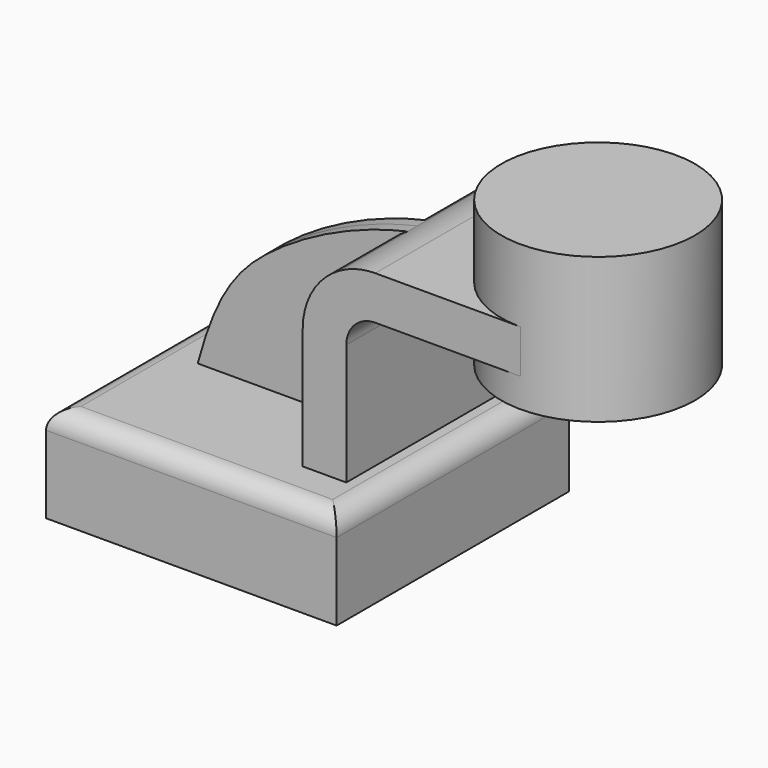
from build123d import *

# Parameters (mm, degrees)
F1_DEPTH = 38.1
F2_DEPTH = 25.4
F4_DEPTH = 3.175
F5_R     = 5.08


with BuildPart() as f1:
    # F0 (on Front) → F1 (new body, symmetric)
    with BuildSketch(Plane.XZ):
        Polygon((38.1, -12.7), (38.1, 12.7), (30.48, 12.7), (19.05, 12.7), (-26.270797, 12.7), (-38.1, 12.7), (-38.1, -12.7), align=None)
    extrude(amount=F1_DEPTH, both=True)

    # F0 (on Front) → F2 (join, symmetric)
    with BuildSketch(Plane.XZ):
        with BuildLine():
            Line((19.05, 12.7), (30.48, 12.7))
            Line((30.48, 12.7), (30.48, 44.45))
            ThreePointArc((30.48, 44.45), (32.711846, 49.838154), (38.1, 52.07))
            Line((38.1, 52.07), (76.2, 52.07))
            Line((76.2, 52.07), (76.2, 63.5))
            Line((76.2, 63.5), (38.1, 63.5))
            ThreePointArc((38.1, 63.5), (33.288873, 62.882459), (28.78967, 61.069875))
            ThreePointArc((28.78967, 61.069875), (21.664303, 54.081737), (19.05, 44.45))
            Line((19.05, 44.45), (19.05, 12.7))
        make_face()
    extrude(amount=F2_DEPTH, both=True)

    # F5
    f5_edges = [f1.edges().sort_by_distance(p)[0] for p in [
        (-38.1, 0, 12.7),
        (0, 38.1, 12.7),
        (38.1, 0, 12.7),
        (0, -38.1, 12.7),
    ]]
    fillet(f5_edges, radius=F5_R)


with BuildPart() as f3:
    # F0 (on Front) → F3 (revolve)
    with BuildSketch(Plane.XZ):
        Polygon((76.2, 63.5), (76.2, 52.07), (76.2, 44.45), (101.6, 44.45), (101.6, 82.55), (76.2, 82.55), align=None)
    revolve(axis=Axis((76.2, 0, 63.5), (0, 0, 1)))


with BuildPart() as f4:
    # F0 (on Front) → F4 (new body, symmetric)
    with BuildSketch(Plane.XZ):
        with BuildLine():
            Line((-26.270797, 12.7), (19.05, 12.7))
            Line((19.05, 12.7), (19.05, 44.45))
            ThreePointArc((19.05, 44.45), (21.664303, 54.081737), (28.78967, 61.069875))
            add(Edge.make_bspline(
                [(-26.270797, 12.7), (-21.3065, 31.380937), (-9.413722, 45.883761), (15.026044, 58.004854), (28.78967, 61.069875)],
                knots=[0, 0, 0, 0, 0.498999, 1, 1, 1, 1], degree=3))
        make_face()
    extrude(amount=F4_DEPTH, both=True)


solid = Compound([f1.part, f3.part, f4.part])
